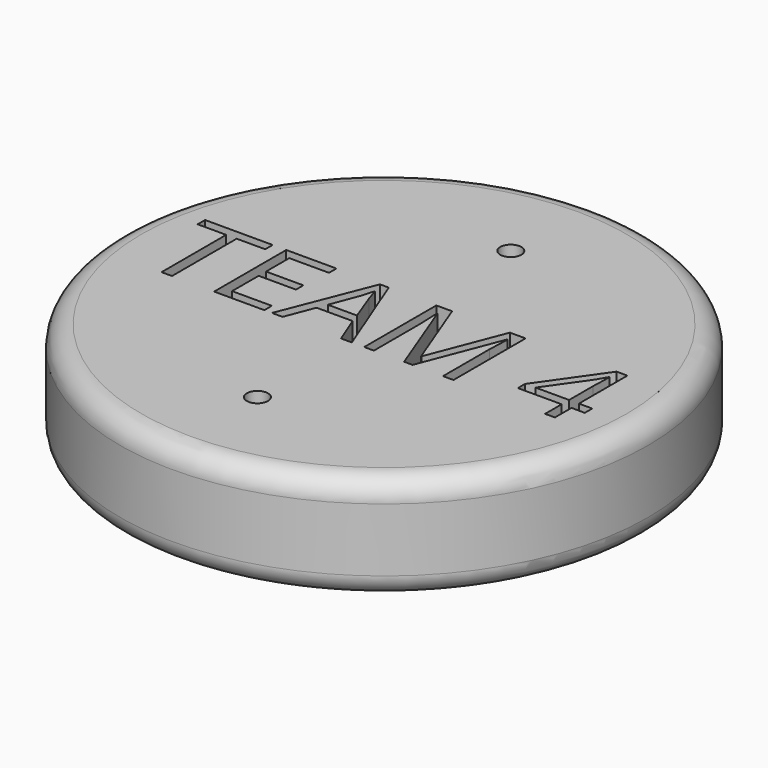
from build123d import *

# Parameters (mm, degrees)
F0_R           = 25
F1_DEPTH       = 10
F2_R           = 2
F4_D           = 2
F4_CBORE_D     = 5
F4_CBORE_DEPTH = 2.5
F5_TEXT_SIZE   = 11.9573954079
F6_DEPTH       = 2.5


# Not quite as in the source:
# - Text() gives the source's letters only with a copy of the font that has no kerning and outlines rounded to 1/6400 em; it was checked with that copy


with BuildPart() as f1:
    # F0 (on Top) → F1 (new body)
    with BuildSketch(Plane.XY):
        Circle(F0_R)
    extrude(amount=F1_DEPTH)

    # F2
    f2_edges = [f1.edges().sort_by_distance(p)[0] for p in [
        (-25, 0, 10),
        (-25, 0, 0),
    ]]
    fillet(f2_edges, radius=F2_R)

    # F4 (through all)
    with Locations(Plane(origin=(0, 0, 0), x_dir=(1, 0, 0), z_dir=(0, 0, -1))):
        with Locations((0, 15), (0, -15)):
            CounterBoreHole(F4_D / 2, F4_CBORE_D / 2, F4_CBORE_DEPTH)

    # F5 (on face) → F6 (cut)
    with BuildSketch(Plane.XY.offset(10)):
        with Locations((-20.8480712026, -3.7982317153)):
            Text('TEAM 4', F5_TEXT_SIZE, font='Open Sans', text_align=(TextAlign.LEFT, TextAlign.BOTTOM))
    extrude(amount=-F6_DEPTH, mode=Mode.SUBTRACT)


solid = f1.part
